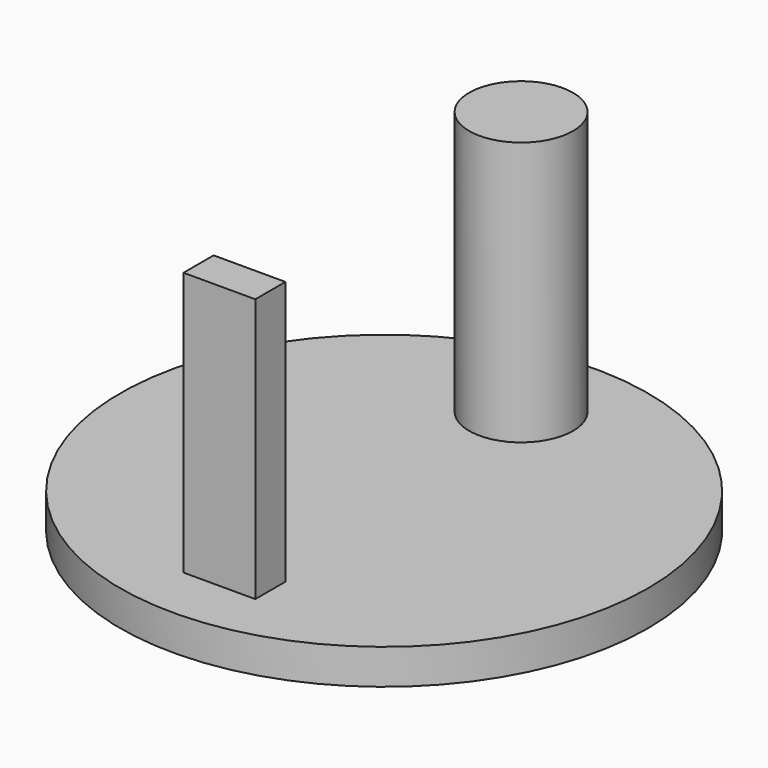
from build123d import *

# Parameters (mm, degrees)
F0_R     = 15
F1_DEPTH = 2
F2_R     = 2.9516544706
F2_W     = 4.0816161782
F2_H     = 2.1391976625
F3_DEPTH = 15


# Not quite as in the source:
# - a feature names something its author has since deleted; it is built from what else it names


with BuildPart() as f1:
    # F0 (on Top) → F1 (new body)
    with BuildSketch(Plane.XY):
        Circle(F0_R)
    extrude(amount=F1_DEPTH)

    # F2 (on face) → F3 (join)
    with BuildSketch(Plane.XY.offset(2)):
        with Locations((0, 9.7299581394)):
            Circle(F2_R)
        with Locations((0, -10.6295719743)):
            Rectangle(F2_W, F2_H)
    extrude(amount=F3_DEPTH)


solid = f1.part
